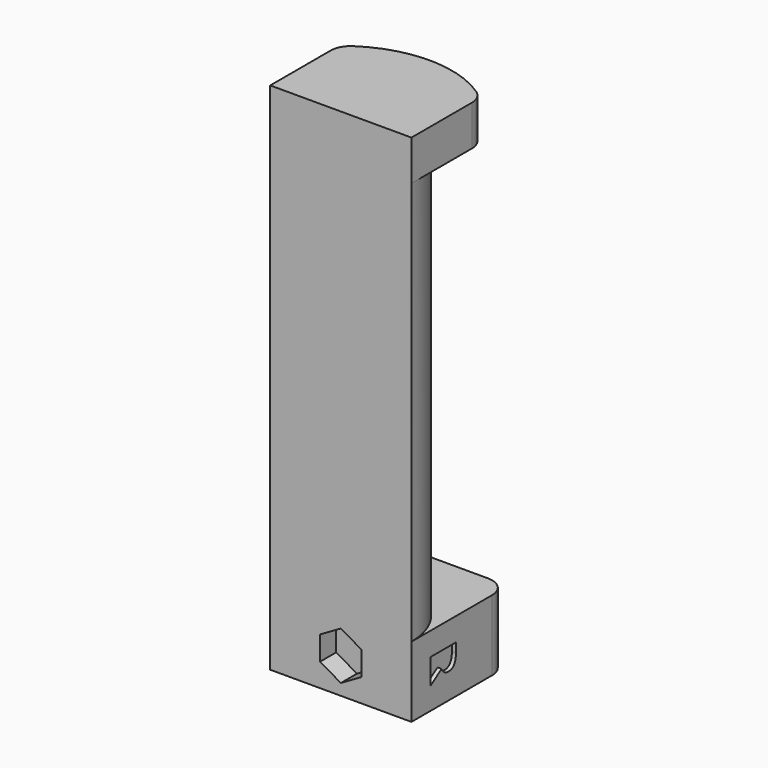
from build123d import *

# Parameters (mm, degrees)
F3_DEPTH     = 8.75
F5_R         = 3.15
F6_DEPTH     = 30
F7_DEPTH     = 5
F9_DEPTH     = 100
F11_DEPTH    = 10
F12_R        = 5
F8_TEXT_SIZE = 11.0344827586
F13_DEPTH    = 1
F14_R        = 3.95
F15_DEPTH    = 0.3


# Not quite as in the source:
# - Text() gives the source's letters only with a copy of the font that has no kerning and outlines rounded to 1/6400 em; it was checked with that copy


with BuildPart() as f3:
    # F2 (on Top) → F3 (new body, symmetric)
    with BuildSketch(Plane.XY):
        with BuildLine():
            ThreePointArc((-17.5, -15), (0, 2.5), (17.5, -15))
            Line((17.5, -15), (17.5, 15))
            Line((17.5, 15), (-17.5, 15))
            Line((-17.5, 15), (-17.5, -15))
        make_face()
        with BuildLine():
            Line((-17.5, -15), (17.5, -15))
            ThreePointArc((17.5, -15), (0, 2.5), (-17.5, -15))
        make_face()
    extrude(amount=F3_DEPTH, both=True)

    # F5 (on face) → F6 (cut, through all)
    with BuildSketch(Plane.XZ.offset(15)):
        Circle(F5_R)
    extrude(amount=-F6_DEPTH, mode=Mode.SUBTRACT)

    # F5 (on face) → F7 (cut)
    with BuildSketch(Plane.XZ.offset(15)):
        Polygon((0, -5.9467077727), (5.15, -2.9733538863), (5.15, 2.9733538863), (0, 5.9467077727), (-5.15, 2.9733538863), (-5.15, -2.9733538863), align=None)
        Circle(F5_R, mode=Mode.SUBTRACT)
    extrude(amount=-F7_DEPTH, mode=Mode.SUBTRACT)

    # F4 (on face) → F9 (join)
    with BuildSketch(Plane.XY.offset(8.75)):
        with BuildLine():
            Line((-17.5, -15), (17.5, -15))
            ThreePointArc((17.5, -15), (0, 2.5), (-17.5, -15))
        make_face()
    extrude(amount=F9_DEPTH)

    # F10 (on face) → F11 (join)
    with BuildSketch(Plane.XY.offset(108.75)):
        with BuildLine():
            Line((17.5, -15), (17.5, 6.2132034356))
            ThreePointArc((17.5, 6.2132034356), (0, 12.5), (-17.5, 6.2132034356))
            Line((-17.5, 6.2132034356), (-17.5, -15))
            ThreePointArc((-17.5, -15), (0, 2.5), (17.5, -15))
        make_face()
        with BuildLine():
            Line((-17.5, -15), (17.5, -15))
            ThreePointArc((17.5, -15), (0, 2.5), (-17.5, -15))
        make_face()
    extrude(amount=F11_DEPTH)

    # F12
    f12_edges = [f3.edges().sort_by_distance(p)[0] for p in [
        (-17.5, 6.213203, 113.75),
        (-17.5, 15, 0),
        (17.5, 15, 0),
        (17.5, 6.213203, 113.75),
    ]]
    fillet(f12_edges, radius=F12_R)

    # F8 (on face) → F13 (cut)
    with BuildSketch(Plane.YZ.offset(17.5)):
        with Locations(Location((-9.1043997179, 4), (0, 0, -90))):
            Text('R', F8_TEXT_SIZE, font='Open Sans', font_style=FontStyle.BOLD, text_align=(TextAlign.LEFT, TextAlign.BOTTOM))
        Polygon((-9.1043997179, 1.3379310345), (-9.1043997179, -1.4310344828), (-6.0819859248, 0.45), (-6.0819859248, 1.3379310345), align=None)
        with BuildLine():
            Line((-2.5957790282, 1.3379310345), (-4.7233652351, 1.3379310345))
            Line((-4.7233652351, 1.3379310345), (-4.7233652351, 0.8))
            add(Edge.make_bspline(
                [(-4.7233652351, 0.8), (-4.7233652351, 0.0068965517), (-4.4595721316, -0.3698275862)],
                knots=[0, 0, 0, 1, 1, 1], degree=2))
            add(Edge.make_bspline(
                [(-4.4595721316, -0.3698275862), (-4.1957790282, -0.7465517241), (-3.6302617868, -0.7465517241)],
                knots=[0, 0, 0, 1, 1, 1], degree=2))
            add(Edge.make_bspline(
                [(-3.6302617868, -0.7465517241), (-3.0699169592, -0.7465517241), (-2.8328479937, -0.3612068966)],
                knots=[0, 0, 0, 1, 1, 1], degree=2))
            add(Edge.make_bspline(
                [(-2.8328479937, -0.3612068966), (-2.5957790282, 0.024137931), (-2.5957790282, 0.8310344828)],
                knots=[0, 0, 0, 1, 1, 1], degree=2))
            Line((-2.5957790282, 0.8310344828), (-2.5957790282, 1.3379310345))
        make_face()
    extrude(amount=-F13_DEPTH, mode=Mode.SUBTRACT)

    # F14 (on face) → F15 (join)
    with BuildSketch(Plane.XZ.offset(10)):
        Circle(F14_R)
    extrude(amount=-F15_DEPTH)


solid = f3.part
